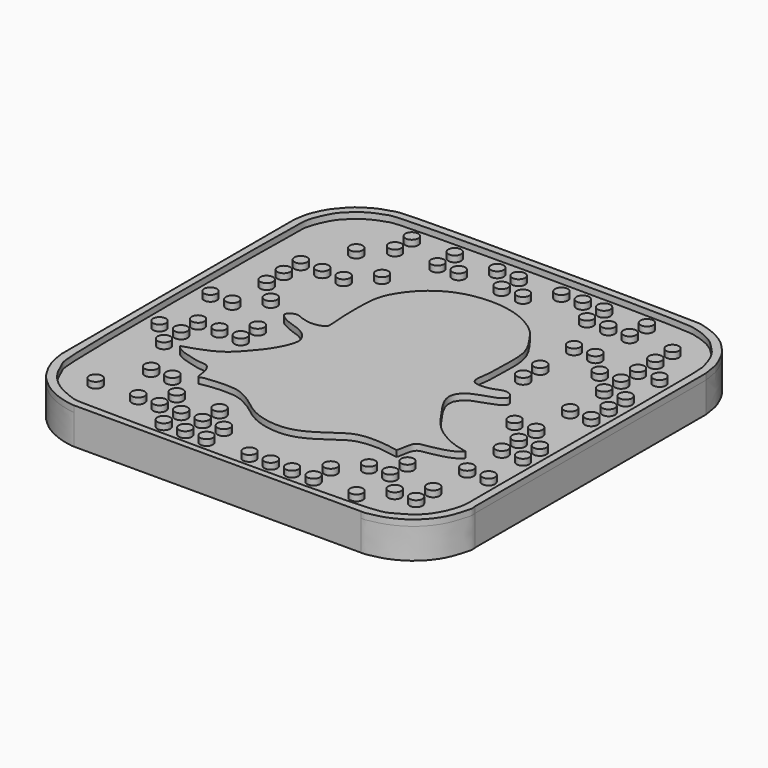
from build123d import *

# Parameters (mm, degrees)
F1_DEPTH = 5
F2_DEPTH = 6
F0_R     = 1.0546287261
F3_DEPTH = 6
F4_DEPTH = 5


with BuildPart() as f1:
    # F0 (on Top) → F1 (new body)
    with BuildSketch(Plane.XY):
        with BuildLine():
            add(Edge.make_bspline(
                [(68.2171358095, 57.8577862937), (68.1561260405, 58.2859510529), (68.0444856387, 59.1366988417), (67.8350567426, 60.3582612354), (67.1676272666, 62.0168375282), (66.397854231, 63.5070858652), (65.2125649418, 64.8392088357), (64.3023803973, 65.7864022985), (62.9966462174, 66.6931312679), (61.3528774809, 67.5070729793), (59.2915900258, 68.120285546), (58.393940965, 68.3472420171), (9.2384246733, 68.7376372657), (8.5465575449, 67.9192863417), (6.7965015741, 67.4906120732), (5.8630514529, 67.0030426438), (4.8075350097, 66.3808713375), (3.5786268933, 65.5566460184), (2.5860120224, 64.2720513708), (1.6983637524, 63.3907617319), (0.5996267097, 61.1541304549), (0.2091955746, 59.7284915791), (0.070267782, 58.6452632175), (0, 58.0973811448)],
                knots=[0, 0, 0, 0, 0.0354924881, 0.0704714419, 0.1121600006, 0.1533957856, 0.1949235555, 0.2309068375, 0.269880155, 0.313649618, 0.3557585841, 0.3964981898, 0.614375585, 0.6532306822, 0.6915842843, 0.7246091785, 0.7588415091, 0.7973073336, 0.8366368413, 0.8723675098, 0.9212086406, 0.9601511273, 1, 1, 1, 1], degree=3))
            add(Edge.make_bspline(
                [(0, 58.0973811448), (0, 42.1047822262), (0, 26.1121833076), (0, 10.119584389)],
                knots=[0, 0, 0, 0, 47.9777967557, 47.9777967557, 47.9777967557, 47.9777967557], degree=3))
            add(Edge.make_bspline(
                [(0, 10.119584389), (0.0191326118, 10.0648531951), (0.0589012098, 9.9510902198), (0.0637936017, 9.7368078743), (0.1167196654, 9.4273162015), (0.1980332736, 8.8210631542), (0.3057776258, 8.4076825759), (0.4580654813, 7.7426581106), (0.6933247773, 7.0445218379), (1.1415628088, 5.9759062805), (1.7829839185, 4.8811749408), (2.6302110043, 3.641757604), (4.0052876158, 2.4562801367), (4.9295718984, 1.7329826728), (6.6153040643, 0.851039242), (8.2478725261, 0.2928080191), (9.901482358, -0.0267490874), (10.1681575885, -0.0062332065), (10.2491797879, 0)],
                knots=[0, 0, 0, 0, 0.0279619861, 0.0581211282, 0.0958969447, 0.1478020137, 0.1924403197, 0.246414422, 0.3043064604, 0.3757396047, 0.4512143282, 0.5337876447, 0.6228800605, 0.6961179759, 0.7865289832, 0.8783792777, 0.9630487676, 1, 1, 1, 1], degree=3))
            add(Edge.make_bspline(
                [(10.2491797879, 0), (26.0407682508, 0), (41.8312546043, 0), (57.6228430672, 0)],
                knots=[0, 0, 0, 0, 47.3736632792, 47.3736632792, 47.3736632792, 47.3736632792], degree=3))
            add(Edge.make_bspline(
                [(57.6228430672, 0), (57.8216606542, -0.0124964305), (58.2520349361, -0.0395149082), (59.0569193754, 0.1931555119), (60.0229768594, 0.3584745814), (61.5223297257, 0.7800704539), (63.6883904749, 1.8829382233), (65.7482479693, 3.6883095056), (67.3823425006, 6.1787406953), (67.9602644801, 8.5638260331), (68.3051873171, 9.4332729864), (68.2171359658, 10.0063476561), (68.1836028834, 10.2927462726)],
                knots=[0, 0, 0, 0, 0.0639988229, 0.137639546, 0.2178598261, 0.3187000191, 0.4454771392, 0.5808046934, 0.7227903341, 0.8489697131, 0.925845904, 1, 1, 1, 1], degree=3))
            add(Edge.make_bspline(
                [(68.1836028834, 10.2927462726), (68.2005396159, 33.6414665491), (68.2173316793, 57.6022151451), (68.2171357667, 57.8527050603), (68.2171357611, 57.8570277108), (68.2171358296, 57.8577862937)],
                knots=[0, 0, 0, 0, 0.9667755289, 0.9916227956, 0.9972307922, 0.9972307922, 0.9972307922, 0.9972307922], degree=3))
        make_face()
        with BuildLine():
            add(Edge.make_bspline(
                [(1.3141017407, 58.6452632175), (1.3031355507, 58.5294157648), (1.3110949493, 58.3599269087), (1.1508208547, 58.1599343384), (0.8378648131, 9.0700756026), (1.8271417922, 8.2208250892), (2.6890632542, 5.8836506349), (4.2017236024, 3.9797285089), (6.0829516081, 2.5606728628), (9.1466977334, 1.2821029614), (11.0679741714, 1.1739902481), (58.8352815393, 0.6597895748), (60.876604208, 2.1021596647), (63.9477454095, 3.6142173707), (65.9633186504, 6.4463741883), (66.9954230728, 9.6963250571), (66.7310188195, 12.2602792173), (67.2463994777, 58.193251624), (66.6936589023, 59.3306298005), (66.046075224, 61.5802917188), (65.0051288779, 63.2158709654), (63.6282950837, 64.4856915447), (63.0746310658, 65.0832489931), (61.9148193122, 65.7932732952), (60.4968537722, 66.3873046431), (59.3003695815, 66.6460938675), (58.3626625451, 67.3329664355), (9.3305644305, 67.3932001844), (8.7036721102, 66.6717789485), (7.1998643305, 66.2413292439), (5.9137335791, 65.5458722903), (4.9628674917, 64.9425428551), (4.1562582814, 64.102559029), (3.15568103, 63.2061280533), (2.2632332671, 61.6115390211), (1.5531488748, 59.8674076777), (1.3378973243, 58.8966411107), (1.3141017407, 58.6452632175)],
                knots=[0, 0, 0, 0, 0.0072201526, 0.0152897887, 0.1166762211, 0.1378771368, 0.1588577716, 0.1817687417, 0.2046070283, 0.22909343, 0.2534755274, 0.3533096535, 0.3789902704, 0.4038605994, 0.4314967269, 0.4561364886, 0.4838383309, 0.5818211398, 0.6011577407, 0.6217100785, 0.6427837553, 0.6623378791, 0.6754775967, 0.6922421281, 0.7107937502, 0.7252413967, 0.7433566321, 0.8448007979, 0.8615172511, 0.8782173334, 0.8962466605, 0.911650917, 0.9271985651, 0.9440254417, 0.9637875706, 0.9843329593, 1, 1, 1, 1], degree=3))
        make_face(mode=Mode.SUBTRACT)
    extrude(amount=F1_DEPTH)

    # F0 (on Top) → F2 (join)
    with BuildSketch(Plane.XY):
        with BuildLine():
            add(Edge.make_bspline(
                [(68.2171358095, 57.8577862937), (68.1561260405, 58.2859510529), (68.0444856387, 59.1366988417), (67.8350567426, 60.3582612354), (67.1676272666, 62.0168375282), (66.397854231, 63.5070858652), (65.2125649418, 64.8392088357), (64.3023803973, 65.7864022985), (62.9966462174, 66.6931312679), (61.3528774809, 67.5070729793), (59.2915900258, 68.120285546), (58.393940965, 68.3472420171), (9.2384246733, 68.7376372657), (8.5465575449, 67.9192863417), (6.7965015741, 67.4906120732), (5.8630514529, 67.0030426438), (4.8075350097, 66.3808713375), (3.5786268933, 65.5566460184), (2.5860120224, 64.2720513708), (1.6983637524, 63.3907617319), (0.5996267097, 61.1541304549), (0.2091955746, 59.7284915791), (0.070267782, 58.6452632175), (0, 58.0973811448)],
                knots=[0, 0, 0, 0, 0.0354924881, 0.0704714419, 0.1121600006, 0.1533957856, 0.1949235555, 0.2309068375, 0.269880155, 0.313649618, 0.3557585841, 0.3964981898, 0.614375585, 0.6532306822, 0.6915842843, 0.7246091785, 0.7588415091, 0.7973073336, 0.8366368413, 0.8723675098, 0.9212086406, 0.9601511273, 1, 1, 1, 1], degree=3))
            add(Edge.make_bspline(
                [(0, 58.0973811448), (0, 42.1047822262), (0, 26.1121833076), (0, 10.119584389)],
                knots=[0, 0, 0, 0, 47.9777967557, 47.9777967557, 47.9777967557, 47.9777967557], degree=3))
            add(Edge.make_bspline(
                [(0, 10.119584389), (0.0191326118, 10.0648531951), (0.0589012098, 9.9510902198), (0.0637936017, 9.7368078743), (0.1167196654, 9.4273162015), (0.1980332736, 8.8210631542), (0.3057776258, 8.4076825759), (0.4580654813, 7.7426581106), (0.6933247773, 7.0445218379), (1.1415628088, 5.9759062805), (1.7829839185, 4.8811749408), (2.6302110043, 3.641757604), (4.0052876158, 2.4562801367), (4.9295718984, 1.7329826728), (6.6153040643, 0.851039242), (8.2478725261, 0.2928080191), (9.901482358, -0.0267490874), (10.1681575885, -0.0062332065), (10.2491797879, 0)],
                knots=[0, 0, 0, 0, 0.0279619861, 0.0581211282, 0.0958969447, 0.1478020137, 0.1924403197, 0.246414422, 0.3043064604, 0.3757396047, 0.4512143282, 0.5337876447, 0.6228800605, 0.6961179759, 0.7865289832, 0.8783792777, 0.9630487676, 1, 1, 1, 1], degree=3))
            add(Edge.make_bspline(
                [(10.2491797879, 0), (26.0407682508, 0), (41.8312546043, 0), (57.6228430672, 0)],
                knots=[0, 0, 0, 0, 47.3736632792, 47.3736632792, 47.3736632792, 47.3736632792], degree=3))
            add(Edge.make_bspline(
                [(57.6228430672, 0), (57.8216606542, -0.0124964305), (58.2520349361, -0.0395149082), (59.0569193754, 0.1931555119), (60.0229768594, 0.3584745814), (61.5223297257, 0.7800704539), (63.6883904749, 1.8829382233), (65.7482479693, 3.6883095056), (67.3823425006, 6.1787406953), (67.9602644801, 8.5638260331), (68.3051873171, 9.4332729864), (68.2171359658, 10.0063476561), (68.1836028834, 10.2927462726)],
                knots=[0, 0, 0, 0, 0.0639988229, 0.137639546, 0.2178598261, 0.3187000191, 0.4454771392, 0.5808046934, 0.7227903341, 0.8489697131, 0.925845904, 1, 1, 1, 1], degree=3))
            add(Edge.make_bspline(
                [(68.1836028834, 10.2927462726), (68.2005396159, 33.6414665491), (68.2173316793, 57.6022151451), (68.2171357667, 57.8527050603), (68.2171357611, 57.8570277108), (68.2171358296, 57.8577862937)],
                knots=[0, 0, 0, 0, 0.9667755289, 0.9916227956, 0.9972307922, 0.9972307922, 0.9972307922, 0.9972307922], degree=3))
        make_face()
        with BuildLine():
            add(Edge.make_bspline(
                [(1.3141017407, 58.6452632175), (1.3031355507, 58.5294157648), (1.3110949493, 58.3599269087), (1.1508208547, 58.1599343384), (0.8378648131, 9.0700756026), (1.8271417922, 8.2208250892), (2.6890632542, 5.8836506349), (4.2017236024, 3.9797285089), (6.0829516081, 2.5606728628), (9.1466977334, 1.2821029614), (11.0679741714, 1.1739902481), (58.8352815393, 0.6597895748), (60.876604208, 2.1021596647), (63.9477454095, 3.6142173707), (65.9633186504, 6.4463741883), (66.9954230728, 9.6963250571), (66.7310188195, 12.2602792173), (67.2463994777, 58.193251624), (66.6936589023, 59.3306298005), (66.046075224, 61.5802917188), (65.0051288779, 63.2158709654), (63.6282950837, 64.4856915447), (63.0746310658, 65.0832489931), (61.9148193122, 65.7932732952), (60.4968537722, 66.3873046431), (59.3003695815, 66.6460938675), (58.3626625451, 67.3329664355), (9.3305644305, 67.3932001844), (8.7036721102, 66.6717789485), (7.1998643305, 66.2413292439), (5.9137335791, 65.5458722903), (4.9628674917, 64.9425428551), (4.1562582814, 64.102559029), (3.15568103, 63.2061280533), (2.2632332671, 61.6115390211), (1.5531488748, 59.8674076777), (1.3378973243, 58.8966411107), (1.3141017407, 58.6452632175)],
                knots=[0, 0, 0, 0, 0.0072201526, 0.0152897887, 0.1166762211, 0.1378771368, 0.1588577716, 0.1817687417, 0.2046070283, 0.22909343, 0.2534755274, 0.3533096535, 0.3789902704, 0.4038605994, 0.4314967269, 0.4561364886, 0.4838383309, 0.5818211398, 0.6011577407, 0.6217100785, 0.6427837553, 0.6623378791, 0.6754775967, 0.6922421281, 0.7107937502, 0.7252413967, 0.7433566321, 0.8448007979, 0.8615172511, 0.8782173334, 0.8962466605, 0.911650917, 0.9271985651, 0.9440254417, 0.9637875706, 0.9843329593, 1, 1, 1, 1], degree=3))
        make_face(mode=Mode.SUBTRACT)
    extrude(amount=F2_DEPTH)


with BuildPart() as f2:
    # F0 (on Top) → F2, piece 2 (new body)
    with BuildSketch(Plane.XY):
        with BuildLine():
            add(Edge.make_bspline(
                [(43.449871242, 52.5479950011), (43.0129453009, 52.9624389986), (42.0322264392, 53.8926951521), (39.4133788223, 55.3667500203), (36.6500072437, 56.0661450298), (33.839108084, 56.3217897121), (30.5907314425, 55.9002072529), (28.162279221, 55.0198683612), (26.0448232179, 53.7026641447), (24.3335941618, 52.0866278396), (22.7718863135, 49.8610431282), (21.8482015345, 47.6458928854), (21.7197726119, 44.3791383594), (21.7600121731, 40.9419799636), (22.0783256756, 37.9839112644), (21.7998947002, 37.4673357038), (21.0336217073, 37.1558010839), (19.8690305863, 36.9098830567), (18.7147084739, 37.1271202667), (17.5996843807, 37.4508042441), (17.0058572743, 37.8345383541), (16.0702478558, 37.5757466982), (15.7330569247, 37.178486094), (15.5695015565, 36.9857937692)],
                knots=[0, 0, 0, 0, 0.0477385433, 0.1071533764, 0.1654893802, 0.2234541007, 0.2855804943, 0.3411144926, 0.3948652757, 0.4478896908, 0.5042040957, 0.5572550505, 0.6188162773, 0.6855032471, 0.7431464172, 0.7667822102, 0.7968583274, 0.8345862555, 0.8723854847, 0.9092266592, 0.9375708446, 0.9697185702, 1, 1, 1, 1], degree=3))
            add(Edge.make_bspline(
                [(15.5695015565, 36.9857937692), (15.5516657247, 36.8775171293), (15.5072989753, 36.608178273), (16.0992462093, 36.0279266028), (17.8336538669, 35.1944210072), (19.52784302, 34.774964683), (20.7597190683, 33.9472718762), (21.4070337599, 33.0688592101), (21.8807208406, 31.8359172568), (20.497263971, 28.550231332), (18.2840237267, 25.9604488041), (16.4019651988, 23.8333879327), (13.6065061469, 22.4019910621), (11.6535871345, 21.8089727485), (10.6754349545, 21.5119495988)],
                knots=[0, 0, 0, 0, 0.0350400423, 0.0871623366, 0.1723966061, 0.2548061463, 0.3277655438, 0.3900045159, 0.456071434, 0.5686105228, 0.6837862909, 0.7858073235, 0.8927180123, 1, 1, 1, 1], degree=3))
            add(Edge.make_bspline(
                [(10.6754349545, 21.5119495988), (10.6489086831, 21.50467136), (10.5800115069, 21.4857674557), (10.6838479534, 21.2778622363), (10.806293289, 21.1075972756), (11.7020844258, 20.4675972322), (13.2714480764, 20.0616964065), (14.9577929767, 19.5281123305), (16.5676321736, 19.6114537044), (17.0550935728, 18.8154782026), (17.5391590165, 17.9966101758), (17.5797962173, 15.9584311972), (18.2101552889, 16.4098497614), (19.6135488621, 16.5419148861), (21.3148153521, 16.6944165776), (23.4215820949, 16.6697190381), (24.899764872, 16.2411322465), (26.8804378634, 15.1396417577), (28.6514546015, 13.5842461377), (31.4124533958, 12.2258191823), (35.5112829189, 11.8133242585), (38.8415601512, 13.2573976808), (41.7490118188, 15.3633469161), (43.6774303666, 16.6268534392), (47.2729333341, 16.8135683339), (49.3478135167, 16.4260777568), (50.4330806434, 16.2332896143)],
                knots=[0, 0, 0, 0, 0.0086434495, 0.022500623, 0.0375418436, 0.0700925826, 0.1122889085, 0.1563603226, 0.1958543304, 0.2244048512, 0.2580666965, 0.2999506684, 0.3207795657, 0.3591826841, 0.402870686, 0.4494525116, 0.4897789088, 0.537862992, 0.5877624477, 0.6443315429, 0.7092476315, 0.7712430281, 0.8320993086, 0.8810721959, 0.9411049235, 1, 1, 1, 1], degree=3))
            add(Edge.make_bspline(
                [(50.4330806434, 16.2332896143), (50.4746928732, 16.2844334773), (50.5966812522, 16.4343643265), (50.7338947295, 17.3257455845), (50.8762482726, 18.2647854121), (51.2773489589, 19.4086468148), (52.7202022984, 19.5205005168), (53.8131545803, 19.7951953089), (55.9573459599, 20.2130486818), (57.4822420624, 21.1377859205), (57.5670241039, 21.4218508153), (57.5924962759, 21.5071961284)],
                knots=[0, 0, 0, 0, 0.053115557, 0.1557109709, 0.268151844, 0.3820910363, 0.5072288805, 0.6274378503, 0.7940080005, 0.9381111429, 1, 1, 1, 1], degree=3))
            add(Edge.make_bspline(
                [(57.5924962759, 21.5071961284), (57.2324622474, 21.5772404813), (56.4362896264, 21.7321352736), (54.8207469061, 22.2076206998), (51.1390191846, 24.0642448928), (48.5635213787, 27.8377864983), (46.5252371365, 30.7455192103), (46.2722918094, 32.852603268), (47.8581300303, 34.6858995215), (51.2223214297, 35.3794032786), (52.8197473542, 36.4786628389), (52.374886585, 37.4567771336), (51.1810735522, 38.0192880682), (49.9019716156, 37.3567799407), (48.3468879808, 36.9899605249), (46.7183372399, 37.0045199092), (45.9431475649, 37.857893095), (46.4938319288, 40.2351914615), (46.4140514619, 42.8455158811), (46.5997554692, 45.9186300015), (46.1212355229, 49.0436804065), (44.3458060948, 51.2972536146), (43.449871242, 52.5479950011)],
                knots=[0, 0, 0, 0, 0.0355947186, 0.0786606866, 0.1459023248, 0.2190266937, 0.2819635171, 0.3276771388, 0.3770388121, 0.4403617363, 0.4832279486, 0.5131283711, 0.5496202343, 0.5889316126, 0.6322699857, 0.6739338104, 0.705878669, 0.7565087994, 0.8121575456, 0.8706937834, 0.9295108093, 1, 1, 1, 1], degree=3))
        make_face()
    extrude(amount=F2_DEPTH)


with BuildPart() as f3:
    # F0 (on Top) → F3 (new body)
    with BuildSketch(Plane.XY):
        with Locations((18.2307194918, 53.5201691091)):
            Circle(F0_R)
        with Locations((14.7421751171, 49.9739795923)):
            Circle(F0_R)
        with Locations((11.19763311, 49.9934181571)):
            Circle(F0_R)
        with Locations((7.6650329866, 49.9934181571)):
            Circle(F0_R)
        with Locations((7.6650329866, 46.4795865119)):
            Circle(F0_R)
        with Locations((7.6650329866, 42.9422520101)):
            Circle(F0_R)
        with Locations((11.19763311, 39.3783077598)):
            Circle(F0_R)
        with Locations((11.1786052585, 57.0336245)):
            Circle(F0_R)
        with Locations((14.7147290409, 60.5879500508)):
            Circle(F0_R)
        with Locations((14.6974250674, 64.0859231353)):
            Circle(F0_R)
        with Locations((21.763605997, 64.1053915024)):
            Circle(F0_R)
        with Locations((21.7872858047, 60.5215616524)):
            Circle(F0_R)
        with Locations((25.2949073911, 60.5215616524)):
            Circle(F0_R)
        with Locations((28.8098808378, 64.0677809715)):
            Circle(F0_R)
        with Locations((32.3377251625, 64.0677809715)):
            Circle(F0_R)
        with Locations((32.3377251625, 60.5632923543)):
            Circle(F0_R)
        with Locations((35.8649156988, 60.5632923543)):
            Circle(F0_R)
        with Locations((39.3852591515, 64.0823319554)):
            Circle(F0_R)
        with Locations((42.9177060723, 64.0823319554)):
            Circle(F0_R)
        with Locations((46.4237891138, 64.0823319554)):
            Circle(F0_R)
        with Locations((46.4237891138, 60.5632923543)):
            Circle(F0_R)
        with Locations((49.9428324401, 60.5632923543)):
            Circle(F0_R)
        with Locations((53.4709133208, 60.5632923543)):
            Circle(F0_R)
        with Locations((53.4709133208, 64.1025975347)):
            Circle(F0_R)
        with Locations((60.5304315686, 60.5632923543)):
            Circle(F0_R)
        with Locations((60.5304315686, 57.0368431509)):
            Circle(F0_R)
        with Locations((53.4902513027, 53.4560009837)):
            Circle(F0_R)
        with Locations((49.9701611698, 53.4560009837)):
            Circle(F0_R)
        with Locations((60.5304315686, 53.4560009837)):
            Circle(F0_R)
        with Locations((64.0808641911, 53.4560009837)):
            Circle(F0_R)
        with Locations((60.5304315686, 49.9584898353)):
            Circle(F0_R)
        with Locations((57.0050738752, 49.9584898353)):
            Circle(F0_R)
        with Locations((60.5304315686, 46.4631132782)):
            Circle(F0_R)
        with Locations((64.0727728605, 46.4631132782)):
            Circle(F0_R)
        with Locations((64.0727728605, 42.9569408298)):
            Circle(F0_R)
        with Locations((64.0727728605, 39.3957793713)):
            Circle(F0_R)
        with Locations((60.5759248137, 39.3957793713)):
            Circle(F0_R)
        with Locations((49.9803349376, 42.9569408298)):
            Circle(F0_R)
        with Locations((49.97510463, 46.4631132782)):
            Circle(F0_R)
        with Locations((57.0098161697, 32.3880128562)):
            Circle(F0_R)
        with Locations((60.5759248137, 32.3880128562)):
            Circle(F0_R)
        with Locations((60.5759248137, 28.7955403328)):
            Circle(F0_R)
        with Locations((64.0665516257, 28.7955403328)):
            Circle(F0_R)
        with Locations((64.0644431114, 25.3155399114)):
            Circle(F0_R)
        with Locations((60.5759248137, 25.3155399114)):
            Circle(F0_R)
        with Locations((60.5434663594, 18.2213000953)):
            Circle(F0_R)
        with Locations((64.0644431114, 18.2213000953)):
            Circle(F0_R)
        with Locations((60.5434663594, 11.1879287288)):
            Circle(F0_R)
        with Locations((60.5434663594, 7.6620965265)):
            Circle(F0_R)
        with Locations((57.0128858089, 7.6620965265)):
            Circle(F0_R)
        with Locations((53.4844063222, 11.1879287288)):
            Circle(F0_R)
        with Locations((53.4844063222, 14.7183416411)):
            Circle(F0_R)
        with Locations((49.9535277486, 11.1879287288)):
            Circle(F0_R)
        with Locations((46.4605391026, 7.6620965265)):
            Circle(F0_R)
        with Locations((46.4605391026, 4.1291620582)):
            Circle(F0_R)
        with Locations((53.5349436104, 4.1291620582)):
            Circle(F0_R)
        with Locations((42.897682637, 4.1291620582)):
            Circle(F0_R)
        with Locations((39.3951125443, 4.1291620582)):
            Circle(F0_R)
        with Locations((35.8751825988, 4.1291620582)):
            Circle(F0_R)
        with Locations((28.8029946387, 4.1195256636)):
            Circle(F0_R)
        with Locations((28.8029946387, 7.6929768547)):
            Circle(F0_R)
        with Locations((25.3010243177, 7.6929768547)):
            Circle(F0_R)
        with Locations((25.3010243177, 11.1886262894)):
            Circle(F0_R)
        with Locations((25.3010243177, 4.1195256636)):
            Circle(F0_R)
        with Locations((21.7513032258, 4.1195256636)):
            Circle(F0_R)
        with Locations((21.7513032258, 7.6929768547)):
            Circle(F0_R)
        with Locations((18.198762089, 7.6929768547)):
            Circle(F0_R)
        with Locations((14.6780563518, 7.6929768547)):
            Circle(F0_R)
        with Locations((18.198762089, 11.2189659849)):
            Circle(F0_R)
        with Locations((7.6572163962, 7.6929768547)):
            Circle(F0_R)
        with Locations((11.1928675324, 14.6939326078)):
            Circle(F0_R)
        with Locations((14.7135742009, 14.6939326078)):
            Circle(F0_R)
        with Locations((7.6650329866, 21.7724423856)):
            Circle(F0_R)
        with Locations((7.6650329866, 25.2907779068)):
            Circle(F0_R)
        with Locations((4.1063698009, 25.2907779068)):
            Circle(F0_R)
        with Locations((7.6650329866, 28.7943482399)):
            Circle(F0_R)
        with Locations((11.2059209496, 28.7943482399)):
            Circle(F0_R)
        with Locations((14.7270234302, 28.7943482399)):
            Circle(F0_R)
        with Locations((14.7270234302, 32.2957932949)):
            Circle(F0_R)
        with Locations((7.6650329866, 35.8634516597)):
            Circle(F0_R)
        with Locations((4.0571894497, 35.8634516597)):
            Circle(F0_R)
    extrude(amount=F3_DEPTH)


with BuildPart() as f4:
    # F0 (on Top) → F4 (new body)
    with BuildSketch(Plane.XY):
        with BuildLine():
            add(Edge.make_bspline(
                [(1.3141017407, 58.6452632175), (1.3031355507, 58.5294157648), (1.3110949493, 58.3599269087), (1.1508208547, 58.1599343384), (0.8378648131, 9.0700756026), (1.8271417922, 8.2208250892), (2.6890632542, 5.8836506349), (4.2017236024, 3.9797285089), (6.0829516081, 2.5606728628), (9.1466977334, 1.2821029614), (11.0679741714, 1.1739902481), (58.8352815393, 0.6597895748), (60.876604208, 2.1021596647), (63.9477454095, 3.6142173707), (65.9633186504, 6.4463741883), (66.9954230728, 9.6963250571), (66.7310188195, 12.2602792173), (67.2463994777, 58.193251624), (66.6936589023, 59.3306298005), (66.046075224, 61.5802917188), (65.0051288779, 63.2158709654), (63.6282950837, 64.4856915447), (63.0746310658, 65.0832489931), (61.9148193122, 65.7932732952), (60.4968537722, 66.3873046431), (59.3003695815, 66.6460938675), (58.3626625451, 67.3329664355), (9.3305644305, 67.3932001844), (8.7036721102, 66.6717789485), (7.1998643305, 66.2413292439), (5.9137335791, 65.5458722903), (4.9628674917, 64.9425428551), (4.1562582814, 64.102559029), (3.15568103, 63.2061280533), (2.2632332671, 61.6115390211), (1.5531488748, 59.8674076777), (1.3378973243, 58.8966411107), (1.3141017407, 58.6452632175)],
                knots=[0, 0, 0, 0, 0.0072201526, 0.0152897887, 0.1166762211, 0.1378771368, 0.1588577716, 0.1817687417, 0.2046070283, 0.22909343, 0.2534755274, 0.3533096535, 0.3789902704, 0.4038605994, 0.4314967269, 0.4561364886, 0.4838383309, 0.5818211398, 0.6011577407, 0.6217100785, 0.6427837553, 0.6623378791, 0.6754775967, 0.6922421281, 0.7107937502, 0.7252413967, 0.7433566321, 0.8448007979, 0.8615172511, 0.8782173334, 0.8962466605, 0.911650917, 0.9271985651, 0.9440254417, 0.9637875706, 0.9843329593, 1, 1, 1, 1], degree=3))
        make_face()
        with Locations((7.6572163962, 7.6929768547)):
            Circle(F0_R, mode=Mode.SUBTRACT)
        with Locations((14.6780563518, 7.6929768547)):
            Circle(F0_R, mode=Mode.SUBTRACT)
        with Locations((11.1928675324, 14.6939326078)):
            Circle(F0_R, mode=Mode.SUBTRACT)
        with Locations((14.7135742009, 14.6939326078)):
            Circle(F0_R, mode=Mode.SUBTRACT)
        with Locations((21.7513032258, 4.1195256636)):
            Circle(F0_R, mode=Mode.SUBTRACT)
        with Locations((25.3010243177, 4.1195256636)):
            Circle(F0_R, mode=Mode.SUBTRACT)
        with Locations((18.198762089, 7.6929768547)):
            Circle(F0_R, mode=Mode.SUBTRACT)
        with Locations((21.7513032258, 7.6929768547)):
            Circle(F0_R, mode=Mode.SUBTRACT)
        with Locations((25.3010243177, 7.6929768547)):
            Circle(F0_R, mode=Mode.SUBTRACT)
        with Locations((28.8029946387, 4.1195256636)):
            Circle(F0_R, mode=Mode.SUBTRACT)
        with Locations((28.8029946387, 7.6929768547)):
            Circle(F0_R, mode=Mode.SUBTRACT)
        with Locations((18.198762089, 11.2189659849)):
            Circle(F0_R, mode=Mode.SUBTRACT)
        with Locations((25.3010243177, 11.1886262894)):
            Circle(F0_R, mode=Mode.SUBTRACT)
        with Locations((4.1063698009, 25.2907779068)):
            Circle(F0_R, mode=Mode.SUBTRACT)
        with Locations((7.6650329866, 21.7724423856)):
            Circle(F0_R, mode=Mode.SUBTRACT)
        with Locations((7.6650329866, 25.2907779068)):
            Circle(F0_R, mode=Mode.SUBTRACT)
        with BuildLine():
            add(Edge.make_bspline(
                [(16.1181768906, 18.3551780309), (16.121574135, 18.3507377643), (16.1249840251, 18.3462809695), (16.1284052418, 18.3417802683)],
                knots=[0, 0, 0, 0, 0.0017391523, 0.0017391523, 0.0017391523, 0.0017391523], degree=3))
            add(Edge.make_bspline(
                [(16.1181768906, 18.3551780309), (16.1321207848, 18.3568460558), (16.1382582967, 18.3610500018), (16.1284052418, 18.3417802683)],
                knots=[0.9947299879, 0.9947299879, 0.9947299879, 0.9947299879, 0.9989637715, 0.9989637715, 0.9989637715, 0.9989637715], degree=3))
        make_face(mode=Mode.SUBTRACT)
        with Locations((7.6650329866, 28.7943482399)):
            Circle(F0_R, mode=Mode.SUBTRACT)
        with Locations((11.2059209496, 28.7943482399)):
            Circle(F0_R, mode=Mode.SUBTRACT)
        with Locations((14.7270234302, 28.7943482399)):
            Circle(F0_R, mode=Mode.SUBTRACT)
        with Locations((14.7270234302, 32.2957932949)):
            Circle(F0_R, mode=Mode.SUBTRACT)
        with BuildLine():
            add(Edge.make_bspline(
                [(15.5695015565, 36.9857937692), (15.5516657247, 36.8775171293), (15.5072989753, 36.608178273), (16.0992462093, 36.0279266028), (17.8336538669, 35.1944210072), (19.52784302, 34.774964683), (20.7597190683, 33.9472718762), (21.4070337599, 33.0688592101), (21.8807208406, 31.8359172568), (20.497263971, 28.550231332), (18.2840237267, 25.9604488041), (16.4019651988, 23.8333879327), (13.6065061469, 22.4019910621), (11.6535871345, 21.8089727485), (10.6754349545, 21.5119495988)],
                knots=[0, 0, 0, 0, 0.0350400423, 0.0871623366, 0.1723966061, 0.2548061463, 0.3277655438, 0.3900045159, 0.456071434, 0.5686105228, 0.6837862909, 0.7858073235, 0.8927180123, 1, 1, 1, 1], degree=3))
            add(Edge.make_bspline(
                [(43.449871242, 52.5479950011), (43.0129453009, 52.9624389986), (42.0322264392, 53.8926951521), (39.4133788223, 55.3667500203), (36.6500072437, 56.0661450298), (33.839108084, 56.3217897121), (30.5907314425, 55.9002072529), (28.162279221, 55.0198683612), (26.0448232179, 53.7026641447), (24.3335941618, 52.0866278396), (22.7718863135, 49.8610431282), (21.8482015345, 47.6458928854), (21.7197726119, 44.3791383594), (21.7600121731, 40.9419799636), (22.0783256756, 37.9839112644), (21.7998947002, 37.4673357038), (21.0336217073, 37.1558010839), (19.8690305863, 36.9098830567), (18.7147084739, 37.1271202667), (17.5996843807, 37.4508042441), (17.0058572743, 37.8345383541), (16.0702478558, 37.5757466982), (15.7330569247, 37.178486094), (15.5695015565, 36.9857937692)],
                knots=[0, 0, 0, 0, 0.0477385433, 0.1071533764, 0.1654893802, 0.2234541007, 0.2855804943, 0.3411144926, 0.3948652757, 0.4478896908, 0.5042040957, 0.5572550505, 0.6188162773, 0.6855032471, 0.7431464172, 0.7667822102, 0.7968583274, 0.8345862555, 0.8723854847, 0.9092266592, 0.9375708446, 0.9697185702, 1, 1, 1, 1], degree=3))
            add(Edge.make_bspline(
                [(57.5924962759, 21.5071961284), (57.2324622474, 21.5772404813), (56.4362896264, 21.7321352736), (54.8207469061, 22.2076206998), (51.1390191846, 24.0642448928), (48.5635213787, 27.8377864983), (46.5252371365, 30.7455192103), (46.2722918094, 32.852603268), (47.8581300303, 34.6858995215), (51.2223214297, 35.3794032786), (52.8197473542, 36.4786628389), (52.374886585, 37.4567771336), (51.1810735522, 38.0192880682), (49.9019716156, 37.3567799407), (48.3468879808, 36.9899605249), (46.7183372399, 37.0045199092), (45.9431475649, 37.857893095), (46.4938319288, 40.2351914615), (46.4140514619, 42.8455158811), (46.5997554692, 45.9186300015), (46.1212355229, 49.0436804065), (44.3458060948, 51.2972536146), (43.449871242, 52.5479950011)],
                knots=[0, 0, 0, 0, 0.0355947186, 0.0786606866, 0.1459023248, 0.2190266937, 0.2819635171, 0.3276771388, 0.3770388121, 0.4403617363, 0.4832279486, 0.5131283711, 0.5496202343, 0.5889316126, 0.6322699857, 0.6739338104, 0.705878669, 0.7565087994, 0.8121575456, 0.8706937834, 0.9295108093, 1, 1, 1, 1], degree=3))
            add(Edge.make_bspline(
                [(50.4330806434, 16.2332896143), (50.4746928732, 16.2844334773), (50.5966812522, 16.4343643265), (50.7338947295, 17.3257455845), (50.8762482726, 18.2647854121), (51.2773489589, 19.4086468148), (52.7202022984, 19.5205005168), (53.8131545803, 19.7951953089), (55.9573459599, 20.2130486818), (57.4822420624, 21.1377859205), (57.5670241039, 21.4218508153), (57.5924962759, 21.5071961284)],
                knots=[0, 0, 0, 0, 0.053115557, 0.1557109709, 0.268151844, 0.3820910363, 0.5072288805, 0.6274378503, 0.7940080005, 0.9381111429, 1, 1, 1, 1], degree=3))
            add(Edge.make_bspline(
                [(10.6754349545, 21.5119495988), (10.6489086831, 21.50467136), (10.5800115069, 21.4857674557), (10.6838479534, 21.2778622363), (10.806293289, 21.1075972756), (11.7020844258, 20.4675972322), (13.2714480764, 20.0616964065), (14.9577929767, 19.5281123305), (16.5676321736, 19.6114537044), (17.0550935728, 18.8154782026), (17.5391590165, 17.9966101758), (17.5797962173, 15.9584311972), (18.2101552889, 16.4098497614), (19.6135488621, 16.5419148861), (21.3148153521, 16.6944165776), (23.4215820949, 16.6697190381), (24.899764872, 16.2411322465), (26.8804378634, 15.1396417577), (28.6514546015, 13.5842461377), (31.4124533958, 12.2258191823), (35.5112829189, 11.8133242585), (38.8415601512, 13.2573976808), (41.7490118188, 15.3633469161), (43.6774303666, 16.6268534392), (47.2729333341, 16.8135683339), (49.3478135167, 16.4260777568), (50.4330806434, 16.2332896143)],
                knots=[0, 0, 0, 0, 0.0086434495, 0.022500623, 0.0375418436, 0.0700925826, 0.1122889085, 0.1563603226, 0.1958543304, 0.2244048512, 0.2580666965, 0.2999506684, 0.3207795657, 0.3591826841, 0.402870686, 0.4494525116, 0.4897789088, 0.537862992, 0.5877624477, 0.6443315429, 0.7092476315, 0.7712430281, 0.8320993086, 0.8810721959, 0.9411049235, 1, 1, 1, 1], degree=3))
        make_face(mode=Mode.SUBTRACT)
        with Locations((35.8751825988, 4.1291620582)):
            Circle(F0_R, mode=Mode.SUBTRACT)
        with Locations((39.3951125443, 4.1291620582)):
            Circle(F0_R, mode=Mode.SUBTRACT)
        with Locations((42.897682637, 4.1291620582)):
            Circle(F0_R, mode=Mode.SUBTRACT)
        with Locations((46.4605391026, 4.1291620582)):
            Circle(F0_R, mode=Mode.SUBTRACT)
        with Locations((46.4605391026, 7.6620965265)):
            Circle(F0_R, mode=Mode.SUBTRACT)
        with Locations((49.9535277486, 11.1879287288)):
            Circle(F0_R, mode=Mode.SUBTRACT)
        with Locations((53.5349436104, 4.1291620582)):
            Circle(F0_R, mode=Mode.SUBTRACT)
        with Locations((57.0128858089, 7.6620965265)):
            Circle(F0_R, mode=Mode.SUBTRACT)
        with Locations((60.5434663594, 7.6620965265)):
            Circle(F0_R, mode=Mode.SUBTRACT)
        with Locations((53.4844063222, 11.1879287288)):
            Circle(F0_R, mode=Mode.SUBTRACT)
        with Locations((53.4844063222, 14.7183416411)):
            Circle(F0_R, mode=Mode.SUBTRACT)
        with Locations((60.5434663594, 11.1879287288)):
            Circle(F0_R, mode=Mode.SUBTRACT)
        with Locations((60.5434663594, 18.2213000953)):
            Circle(F0_R, mode=Mode.SUBTRACT)
        with Locations((64.0644431114, 18.2213000953)):
            Circle(F0_R, mode=Mode.SUBTRACT)
        with Locations((60.5759248137, 25.3155399114)):
            Circle(F0_R, mode=Mode.SUBTRACT)
        with Locations((64.0644431114, 25.3155399114)):
            Circle(F0_R, mode=Mode.SUBTRACT)
        with Locations((57.0098161697, 32.3880128562)):
            Circle(F0_R, mode=Mode.SUBTRACT)
        with Locations((60.5759248137, 28.7955403328)):
            Circle(F0_R, mode=Mode.SUBTRACT)
        with Locations((64.0665516257, 28.7955403328)):
            Circle(F0_R, mode=Mode.SUBTRACT)
        with Locations((60.5759248137, 32.3880128562)):
            Circle(F0_R, mode=Mode.SUBTRACT)
        with Locations((4.0571894497, 35.8634516597)):
            Circle(F0_R, mode=Mode.SUBTRACT)
        with Locations((7.6650329866, 35.8634516597)):
            Circle(F0_R, mode=Mode.SUBTRACT)
        with Locations((7.6650329866, 42.9422520101)):
            Circle(F0_R, mode=Mode.SUBTRACT)
        with Locations((11.19763311, 39.3783077598)):
            Circle(F0_R, mode=Mode.SUBTRACT)
        with Locations((7.6650329866, 46.4795865119)):
            Circle(F0_R, mode=Mode.SUBTRACT)
        with Locations((7.6650329866, 49.9934181571)):
            Circle(F0_R, mode=Mode.SUBTRACT)
        with Locations((11.19763311, 49.9934181571)):
            Circle(F0_R, mode=Mode.SUBTRACT)
        with Locations((14.7421751171, 49.9739795923)):
            Circle(F0_R, mode=Mode.SUBTRACT)
        with Locations((11.1786052585, 57.0336245)):
            Circle(F0_R, mode=Mode.SUBTRACT)
        with Locations((14.7147290409, 60.5879500508)):
            Circle(F0_R, mode=Mode.SUBTRACT)
        with Locations((14.6974250674, 64.0859231353)):
            Circle(F0_R, mode=Mode.SUBTRACT)
        with Locations((18.2307194918, 53.5201691091)):
            Circle(F0_R, mode=Mode.SUBTRACT)
        with Locations((21.7872858047, 60.5215616524)):
            Circle(F0_R, mode=Mode.SUBTRACT)
        with Locations((25.2949073911, 60.5215616524)):
            Circle(F0_R, mode=Mode.SUBTRACT)
        with Locations((21.763605997, 64.1053915024)):
            Circle(F0_R, mode=Mode.SUBTRACT)
        with Locations((28.8098808378, 64.0677809715)):
            Circle(F0_R, mode=Mode.SUBTRACT)
        with Locations((32.3377251625, 60.5632923543)):
            Circle(F0_R, mode=Mode.SUBTRACT)
        with Locations((32.3377251625, 64.0677809715)):
            Circle(F0_R, mode=Mode.SUBTRACT)
        with Locations((49.9803349376, 42.9569408298)):
            Circle(F0_R, mode=Mode.SUBTRACT)
        with Locations((49.97510463, 46.4631132782)):
            Circle(F0_R, mode=Mode.SUBTRACT)
        with Locations((60.5759248137, 39.3957793713)):
            Circle(F0_R, mode=Mode.SUBTRACT)
        with Locations((64.0727728605, 39.3957793713)):
            Circle(F0_R, mode=Mode.SUBTRACT)
        with Locations((57.0050738752, 49.9584898353)):
            Circle(F0_R, mode=Mode.SUBTRACT)
        with Locations((60.5304315686, 46.4631132782)):
            Circle(F0_R, mode=Mode.SUBTRACT)
        with Locations((64.0727728605, 42.9569408298)):
            Circle(F0_R, mode=Mode.SUBTRACT)
        with Locations((64.0727728605, 46.4631132782)):
            Circle(F0_R, mode=Mode.SUBTRACT)
        with Locations((60.5304315686, 49.9584898353)):
            Circle(F0_R, mode=Mode.SUBTRACT)
        with Locations((49.9701611698, 53.4560009837)):
            Circle(F0_R, mode=Mode.SUBTRACT)
        with Locations((35.8649156988, 60.5632923543)):
            Circle(F0_R, mode=Mode.SUBTRACT)
        with Locations((39.3852591515, 64.0823319554)):
            Circle(F0_R, mode=Mode.SUBTRACT)
        with Locations((46.4237891138, 60.5632923543)):
            Circle(F0_R, mode=Mode.SUBTRACT)
        with Locations((42.9177060723, 64.0823319554)):
            Circle(F0_R, mode=Mode.SUBTRACT)
        with Locations((46.4237891138, 64.0823319554)):
            Circle(F0_R, mode=Mode.SUBTRACT)
        with Locations((49.9428324401, 60.5632923543)):
            Circle(F0_R, mode=Mode.SUBTRACT)
        with Locations((53.4902513027, 53.4560009837)):
            Circle(F0_R, mode=Mode.SUBTRACT)
        with Locations((60.5304315686, 53.4560009837)):
            Circle(F0_R, mode=Mode.SUBTRACT)
        with Locations((64.0808641911, 53.4560009837)):
            Circle(F0_R, mode=Mode.SUBTRACT)
        with Locations((60.5304315686, 57.0368431509)):
            Circle(F0_R, mode=Mode.SUBTRACT)
        with Locations((53.4709133208, 60.5632923543)):
            Circle(F0_R, mode=Mode.SUBTRACT)
        with Locations((53.4709133208, 64.1025975347)):
            Circle(F0_R, mode=Mode.SUBTRACT)
        with Locations((60.5304315686, 60.5632923543)):
            Circle(F0_R, mode=Mode.SUBTRACT)
    extrude(amount=F4_DEPTH)


solid = Compound([f1.part, f2.part, f3.part, f4.part])
